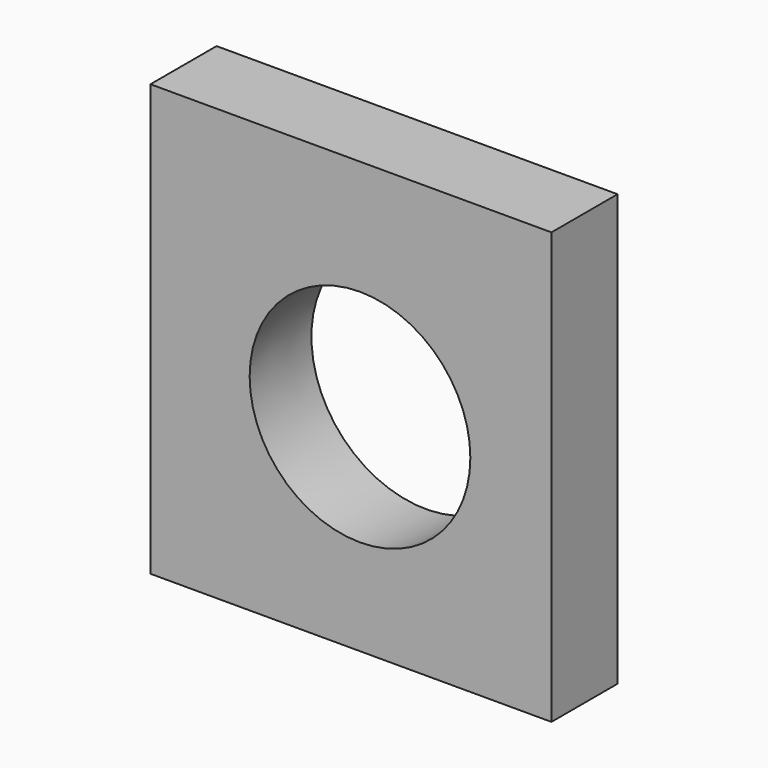
from build123d import *

# Parameters (mm, degrees)
F0_W     = 123.2844814658
F0_H     = 132.5032711029
F1_DEPTH = 25.4
F2_R     = 33.9258484302
F3_DEPTH = 25.4
F3_TAPER = -3


with BuildPart() as f1:
    # F0 (on Front) → F1 (new body)
    with BuildSketch(Plane.XZ):
        with Locations((-162.3135991395, -66.2516355515)):
            Rectangle(F0_W, F0_H)
    extrude(amount=F1_DEPTH)

    # F2 (on face) → F3 (cut)
    with BuildSketch(Plane.XZ.offset(25.4)):
        with Locations((-159.5336198807, -69.13626194)):
            Circle(F2_R)
    extrude(amount=-F3_DEPTH, taper=F3_TAPER, mode=Mode.SUBTRACT)


solid = f1.part
